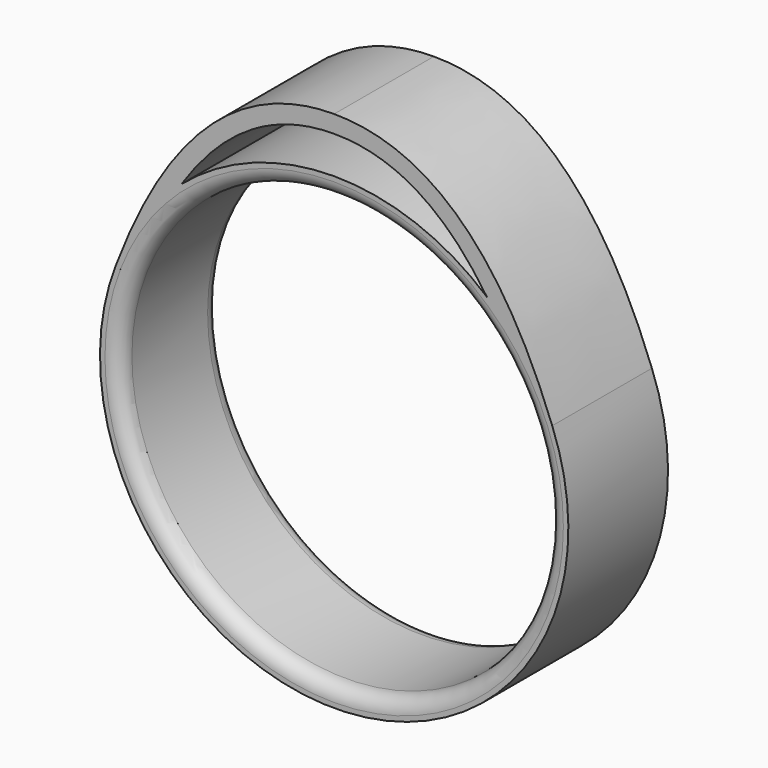
from build123d import *

# Parameters (mm, degrees)
F0_R     = 9.4
F0_R_2   = 8.6
F1_DEPTH = 5
F3_DEPTH = 5
F4_R     = 0.6


# Not quite as in the source:
# - the dataset's text gives a spline's control points without its knots; the knots are read off the source's solid


with BuildPart() as f1:
    # F0 (on Front) → F1 (new body)
    with BuildSketch(Plane.XZ):
        Circle(F0_R)
        Circle(F0_R_2, mode=Mode.SUBTRACT)
    extrude(amount=F1_DEPTH)

    # F2 (on Front) → F3 (join)
    with BuildSketch(Plane.XZ):
        with BuildLine():
            add(Edge.make_bspline(
                [(-8.8490276873, 3.1709161121), (-7.3496829409, 7.2272375548), (-4.746891386, 11.5964177027), (3.78631e-05, 11.5964002776), (5.67948e-05, 11.5964002775)],
                knots=[0, 0, 0, 0, 0.5, 0.5000019941, 0.5000019941, 0.5000019941, 0.5000019941], degree=3))
            Line((-8.8490276873, 3.1709161121), (-8.1924457198, 2.9282226429))
            add(Edge.make_bspline(
                [(-8.1924457198, 2.9282226429), (-7.8262756691, 3.9188576733), (-6.9626502108, 5.9278467604), (-5.4967702335, 8.1305819439), (-4.0755610615, 9.4931807293), (-2.8820227839, 10.2720641504), (-1.7694285607, 10.6893985819), (-0.7912754674, 10.8653850416), (-0.2703531008, 10.896417707), (0, 10.8964002777)],
                knots=[0, 0, 0, 0, 0.125, 0.25, 0.3125, 0.375, 0.4375, 0.46875, 0.5, 0.5, 0.5, 0.5], degree=3))
            add(Edge.make_bspline(
                [(8.1924457198, 2.9282226429), (7.8262756691, 3.9188576733), (6.9626502108, 5.9278467604), (5.4967702335, 8.1305819439), (4.0755610615, 9.4931807293), (2.8820227839, 10.2720641504), (1.7694285607, 10.6893985819), (0.7912754674, 10.8653850416), (0.2703531008, 10.896417707), (0, 10.8964002777)],
                knots=[0, 0, 0, 0, 0.125, 0.25, 0.3125, 0.375, 0.4375, 0.46875, 0.5, 0.5, 0.5, 0.5], degree=3))
            Line((8.1924457198, 2.9282226429), (8.8490276873, 3.1709161121))
            add(Edge.make_bspline(
                [(8.8490276873, 3.1709161121), (7.3496889206, 7.2272213774), (4.7469225273, 11.5963654275), (5.67948e-05, 11.5964002775)],
                knots=[0, 0, 0, 0, 0.4999980059, 0.4999980059, 0.4999980059, 0.4999980059], degree=3))
        make_face()
    extrude(amount=F3_DEPTH)

    # F4
    f4_edges = [f1.edges().sort_by_distance(p)[0] for p in [
        (-8.6, -5, 0),
        (-8.6, 0, 0),
    ]]
    fillet(f4_edges, radius=F4_R)


solid = f1.part
